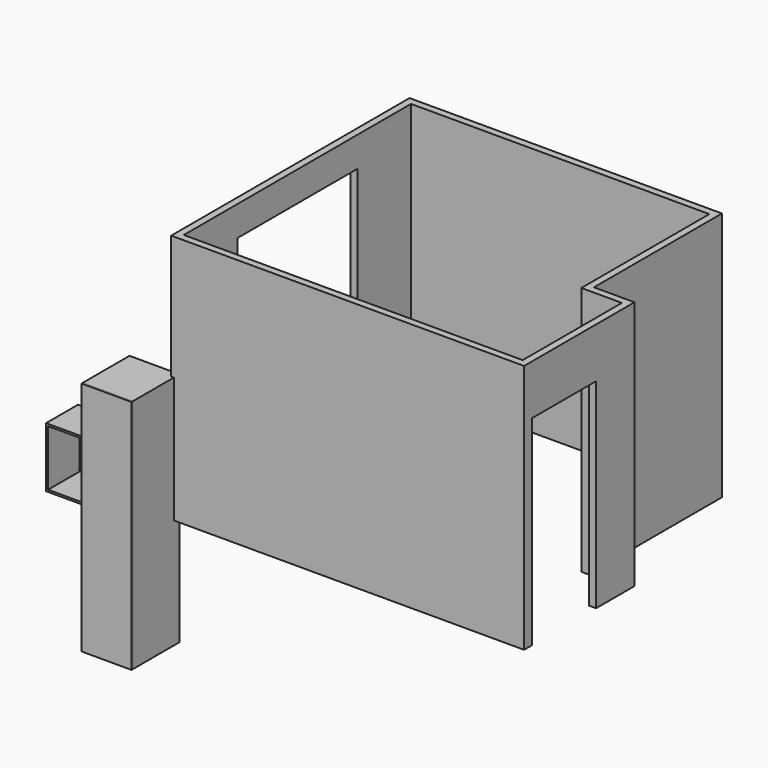
from build123d import *

# Parameters (mm, degrees)
F1_DEPTH  = 2500
F2_W      = 800
F2_H      = 2000
F3_DEPTH  = 70
F4_W      = 1500
F4_H      = 1500
F5_DEPTH  = 70
F6_W      = 500
F6_H      = 2360
F6_W_2    = 460
F6_H_2    = 2320
F7_DEPTH  = 580
F8_W      = 500
F8_H      = 2360
F9_DEPTH  = 5
F10_W     = 500
F10_H     = 2360
F11_DEPTH = 20
F12_W     = 600
F12_H     = 600
F12_W_2   = 560
F12_H_2   = 560
F13_DEPTH = 400
F14_W     = 600
F14_H     = 600
F15_DEPTH = 5


with BuildPart() as f1:
    # F0 (on Top) → F1 (new body)
    with BuildSketch(Plane.XY):
        Polygon((3460, -70), (3460, 830), (3460, 1310), (3055, 1310), (3055, 2910), (-70, 2910), (-70, -70), align=None)
        Polygon((3390, 0), (0, 0), (0, 2840), (2985, 2840), (2985, 1240), (3390, 1240), (3390, 830), align=None, mode=Mode.SUBTRACT)
    extrude(amount=F1_DEPTH)

    # F2 (on face) → F3 (cut, through all)
    with BuildSketch(Plane(origin=(3390, 0, 0), x_dir=(0, -1, 0), z_dir=(-1, 0, 0))):
        with Locations((-430, 1000)):
            Rectangle(F2_W, F2_H)
    extrude(amount=-F3_DEPTH, mode=Mode.SUBTRACT)

    # F4 (on face) → F5 (cut, through all)
    with BuildSketch(Plane.YZ):
        with Locations((1420, 1450)):
            Rectangle(F4_W, F4_H)
    extrude(amount=-F5_DEPTH, mode=Mode.SUBTRACT)


with BuildPart() as f7:
    # F6 (on Front) → F7 (new body)
    with BuildSketch(Plane.XZ):
        with Locations((-293.5058398881, 78.9764812216)):
            Rectangle(F6_W, F6_H)
        with Locations((-293.5058398881, 78.9764812216)):
            Rectangle(F6_W_2, F6_H_2, mode=Mode.SUBTRACT)
    extrude(amount=F7_DEPTH)

    # F8 (on face) → F9 (join)
    with BuildSketch(Plane(origin=(0, 0, 0), x_dir=(-1, 0, 0), z_dir=(0, 1, 0))):
        with Locations((293.5058398881, 78.9764812216)):
            Rectangle(F8_W, F8_H)
    extrude(amount=-F9_DEPTH)


with BuildPart() as f11:
    # F10 (on face) → F11 (new body)
    with BuildSketch(Plane.XZ.offset(580)):
        with Locations((-293.5058398881, 78.9764812216)):
            Rectangle(F10_W, F10_H)
    extrude(amount=F11_DEPTH)


with BuildPart() as f13:
    # F12 (on Front) → F13 (new body)
    with BuildSketch(Plane.XZ):
        with Locations((-758.0079734325, 361.3910255028)):
            Rectangle(F12_W, F12_H)
        with Locations((-758.0079734325, 361.3910255028)):
            Rectangle(F12_W_2, F12_H_2, mode=Mode.SUBTRACT)
    extrude(amount=F13_DEPTH)

    # F14 (on face) → F15 (join)
    with BuildSketch(Plane(origin=(0, 0, 0), x_dir=(-1, 0, 0), z_dir=(0, 1, 0))):
        with Locations((758.0079734325, 361.3910255028)):
            Rectangle(F14_W, F14_H)
    extrude(amount=-F15_DEPTH)


solid = Compound([f1.part, f7.part, f11.part, f13.part])
